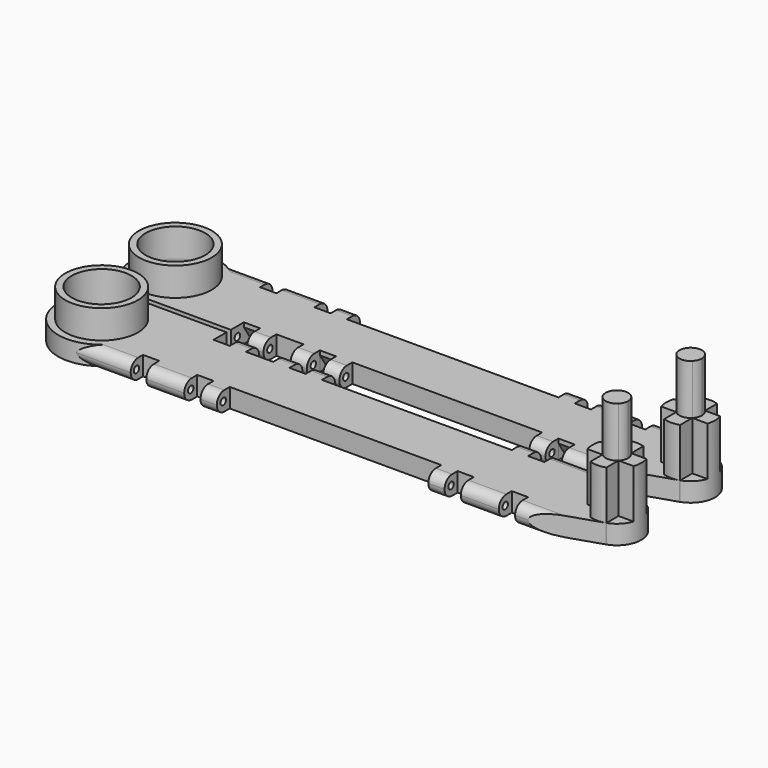
from build123d import *

# Parameters (mm, degrees)
F0_R      = 13.4
F0_R_2    = 11
F0_W      = 6
F0_H      = 6
F1_DEPTH  = 3.5
F2_DEPTH  = 21.5
F3_DEPTH  = 40
F4_DEPTH  = 3.5
F5_R      = 1.25
F6_DEPTH  = 34
F7_DEPTH  = 116
F8_R      = 1.25
F9_DEPTH  = 38
F10_DEPTH = 116
F11_R     = 3.49999
F12_W     = 6
F12_H     = 10
F13_ANGLE = 57
F14_DEPTH = 14


# Not quite as in the source:
# - a fillet or chamfer is up to 0.001 mm smaller than in the source, because OpenCascade refuses the exact size
# - a feature names something its author has since deleted; it is built from what else it names


with BuildPart() as f1:
    # F0 (on Top) → F1 (new body)
    with BuildSketch(Plane.XY):
        with BuildLine():
            ThreePointArc((86.4885738563, -2.925), (86, 0), (86.4885738563, 2.925))
            ThreePointArc((86.4885738563, 2.925), (87.9140641886, 5.5488299377), (90.1195766297, 7.561842879))
            Line((90.1195766297, 7.561842879), (75, 12.5))
            Line((75, 12.5), (73.75, 12.5))
            Line((73.75, 12.5), (73.75, 6.5))
            Line((73.75, 6.5), (-80.3798084828, 6.5))
            ThreePointArc((-80.3798084828, 6.5), (-79.3487530165, 3.3224189775), (-79, 0))
            ThreePointArc((-79, 0), (-80.5812643612, -6.9354208653), (-85.0125078223, -12.5))
            Line((-85.0125078223, -12.5), (-65.25, -12.5))
            Line((-65.25, -12.5), (-65.25, -6.5))
            Line((-65.25, -6.5), (63.75, -6.5))
            Line((63.75, -6.5), (63.75, -12.5))
            Line((63.75, -12.5), (75, -12.5))
            Line((75, -12.5), (90.1195766297, -7.561842879))
            ThreePointArc((90.1195766297, -7.561842879), (87.9140641886, -5.5488299377), (86.4885738563, -2.925))
        make_face()
        with BuildLine():
            ThreePointArc((92.0560443278, 8.5048883003), (94.9210029481, 8.999653297), (97.7942053305, 8.5552566631))
            Line((97.7942053305, 8.5552566631), (75, 16))
            Line((75, 16), (70.25, 16))
            Line((70.25, 16), (70.25, 10))
            Line((70.25, 10), (64.25, 10))
            Line((64.25, 10), (64.25, 16))
            Line((64.25, 16), (50.25, 16))
            Line((50.25, 16), (50.25, 10))
            Line((50.25, 10), (44.25, 10))
            Line((44.25, 10), (44.25, 16))
            Line((44.25, 16), (38.25, 16))
            Line((38.25, 16), (38.25, 10))
            Line((38.25, 10), (-33.75, 10))
            Line((-33.75, 10), (-39.75, 10))
            Line((-39.75, 10), (-39.75, 16))
            Line((-39.75, 16), (-45.75, 16))
            Line((-45.75, 16), (-45.75, 10))
            Line((-45.75, 10), (-51.75, 10))
            Line((-51.75, 10), (-51.75, 16))
            Line((-51.75, 16), (-65.75, 16))
            Line((-65.75, 16), (-65.75, 10))
            Line((-65.75, 10), (-71.75, 10))
            Line((-71.75, 10), (-71.75, 15.6664450339))
            Line((-71.75, 15.6664450339), (-91.75, 15.6664450339))
            ThreePointArc((-91.75, 15.6664450339), (-84.9579949783, 12.4562488392), (-80.3798084828, 6.5))
            Line((-80.3798084828, 6.5), (73.75, 6.5))
            Line((73.75, 6.5), (73.75, 12.5))
            Line((73.75, 12.5), (75, 12.5))
            Line((75, 12.5), (90.1195766297, 7.561842879))
            ThreePointArc((90.1195766297, 7.561842879), (91.0594974284, 8.0915041545), (92.0560443278, 8.5048883003))
        make_face()
        with BuildLine():
            ThreePointArc((-79, 0), (-79.3487530165, 3.3224189775), (-80.3798084828, 6.5))
            ThreePointArc((-80.3798084828, 6.5), (-84.9579949783, 12.4562488392), (-91.75, 15.6664450339))
            ThreePointArc((-91.75, 15.6664450339), (-110.9163928159, 1.6335359588), (-95, -16))
            ThreePointArc((-95, -16), (-89.7084973779, -15.0996688705), (-85.0125078223, -12.5))
            ThreePointArc((-85.0125078223, -12.5), (-80.5812643612, -6.9354208653), (-79, 0))
        make_face()
        with Locations((-95, 0)):
            Circle(F0_R, mode=Mode.SUBTRACT)
        with BuildLine():
            Line((75, -16), (97.7942053305, -8.5552566631))
            ThreePointArc((97.7942053305, -8.5552566631), (94.9210029481, -8.999653297), (92.0560443278, -8.5048883003))
            ThreePointArc((92.0560443278, -8.5048883003), (91.0594974284, -8.0915041545), (90.1195766297, -7.561842879))
            Line((90.1195766297, -7.561842879), (75, -12.5))
            Line((75, -12.5), (63.75, -12.5))
            Line((63.75, -12.5), (63.75, -6.5))
            Line((63.75, -6.5), (-65.25, -6.5))
            Line((-65.25, -6.5), (-65.25, -12.5))
            Line((-65.25, -12.5), (-85.0125078223, -12.5))
            ThreePointArc((-85.0125078223, -12.5), (-89.7084973779, -15.0996688705), (-95, -16))
            Line((-95, -16), (-61.75, -16))
            Line((-61.75, -16), (-61.75, -10))
            Line((-61.75, -10), (-55.75, -10))
            Line((-55.75, -10), (-55.75, -16))
            Line((-55.75, -16), (-49.75, -16))
            Line((-49.75, -16), (-49.75, -10))
            Line((-49.75, -10), (-43.75, -10))
            Line((-43.75, -10), (-39.75, -10))
            Line((-39.75, -10), (-33.75, -10))
            Line((-33.75, -10), (-27.75, -10))
            Line((-27.75, -10), (-21.75, -10))
            Line((-21.75, -10), (48.25, -10))
            Line((48.25, -10), (48.25, -16))
            Line((48.25, -16), (54.25, -16))
            Line((54.25, -16), (54.25, -10))
            Line((54.25, -10), (60.25, -10))
            Line((60.25, -10), (60.25, -16))
            Line((60.25, -16), (75, -16))
        make_face()
        with Locations((-95, 0)):
            Circle(F0_R)
        with Locations((-95, 0)):
            Circle(F0_R_2, mode=Mode.SUBTRACT)
        with Locations((-36.75, -13)):
            Rectangle(F0_W, F0_H)
        with Locations((-24.75, -13)):
            Rectangle(F0_W, F0_H)
        with BuildLine():
            ThreePointArc((90.3422779173, -2.925), (89.5, 0), (90.3422779173, 2.925))
            Line((90.3422779173, 2.925), (86.4885738563, 2.925))
            ThreePointArc((86.4885738563, 2.925), (86, 0), (86.4885738563, -2.925))
            Line((86.4885738563, -2.925), (90.3422779173, -2.925))
        make_face()
        with BuildLine():
            Line((103.5114261437, 2.925), (99.6577220827, 2.925))
            ThreePointArc((99.6577220827, 2.925), (100.285237528, 1.5219278145), (100.5, 0))
            ThreePointArc((100.5, 0), (100.285237528, -1.5219278145), (99.6577220827, -2.925))
            Line((99.6577220827, -2.925), (103.5114261437, -2.925))
            ThreePointArc((103.5114261437, -2.925), (103.8770162581, -1.4827617318), (104, 0))
            ThreePointArc((104, 0), (103.8770162581, 1.4827617318), (103.5114261437, 2.925))
        make_face()
        with BuildLine():
            Line((103.5114261437, -2.925), (99.6577220827, -2.925))
            ThreePointArc((99.6577220827, -2.925), (98.8970031473, -3.8811553009), (97.9439556722, -4.6457641998))
            Line((97.9439556722, -4.6457641998), (97.9439556722, -8.5048883003))
            ThreePointArc((97.9439556722, -8.5048883003), (101.3710463425, -6.3568678216), (103.5114261437, -2.925))
        make_face()
        with BuildLine():
            Line((97.9439556722, 8.5048883003), (97.9439556722, 4.6457641998))
            ThreePointArc((97.9439556722, 4.6457641998), (98.8970031473, 3.8811553009), (99.6577220827, 2.925))
            Line((99.6577220827, 2.925), (103.5114261437, 2.925))
            ThreePointArc((103.5114261437, 2.925), (101.3710463425, 6.3568678216), (97.9439556722, 8.5048883003))
        make_face()
        with BuildLine():
            Line((97.9439556722, -8.5048883003), (97.9439556722, -4.6457641998))
            ThreePointArc((97.9439556722, -4.6457641998), (97.4047291369, -4.9464409203), (96.8352012857, -5.1847889293))
            Line((96.8352012857, -5.1847889293), (92.0560443278, -6.876413239))
            Line((92.0560443278, -6.876413239), (92.0560443278, -8.5048883003))
            ThreePointArc((92.0560443278, -8.5048883003), (94.9210029481, -8.999653297), (97.7942053305, -8.5552566631))
            ThreePointArc((97.7942053305, -8.5552566631), (97.8691910299, -8.5304010945), (97.9439556722, -8.5048883003))
        make_face()
        with BuildLine():
            ThreePointArc((96.8352012857, 5.1847889293), (97.4047291369, 4.9464409203), (97.9439556722, 4.6457641998))
            Line((97.9439556722, 4.6457641998), (97.9439556722, 8.5048883003))
            ThreePointArc((97.9439556722, 8.5048883003), (97.8691910299, 8.5304010945), (97.7942053305, 8.5552566631))
            ThreePointArc((97.7942053305, 8.5552566631), (94.9210029481, 8.999653297), (92.0560443278, 8.5048883003))
            Line((92.0560443278, 8.5048883003), (92.0560443278, 6.876413239))
            Line((92.0560443278, 6.876413239), (96.8352012857, 5.1847889293))
        make_face()
        with BuildLine():
            Line((92.0560443278, -6.876413239), (92.0560443278, -4.6457641998))
            ThreePointArc((92.0560443278, -4.6457641998), (91.1029968527, -3.8811553009), (90.3422779173, -2.925))
            Line((90.3422779173, -2.925), (86.4885738563, -2.925))
            ThreePointArc((86.4885738563, -2.925), (87.9140641886, -5.5488299377), (90.1195766297, -7.561842879))
            Line((90.1195766297, -7.561842879), (92.0560443278, -6.876413239))
        make_face()
        with BuildLine():
            ThreePointArc((90.3422779173, 2.925), (91.1029968527, 3.8811553009), (92.0560443278, 4.6457641998))
            Line((92.0560443278, 4.6457641998), (92.0560443278, 6.876413239))
            Line((92.0560443278, 6.876413239), (90.1195766297, 7.561842879))
            ThreePointArc((90.1195766297, 7.561842879), (87.9140641886, 5.5488299377), (86.4885738563, 2.925))
            Line((86.4885738563, 2.925), (90.3422779173, 2.925))
        make_face()
        with BuildLine():
            Line((97.9439556722, -4.6457641998), (97.9439556722, -2.925))
            ThreePointArc((97.9439556722, -2.925), (95, -4.15), (92.0560443278, -2.925))
            Line((92.0560443278, -2.925), (92.0560443278, -4.6457641998))
            ThreePointArc((92.0560443278, -4.6457641998), (94.3835821327, -5.465348023), (96.8352012857, -5.1847889293))
            ThreePointArc((96.8352012857, -5.1847889293), (97.4047291369, -4.9464409203), (97.9439556722, -4.6457641998))
        make_face()
        with BuildLine():
            ThreePointArc((92.0560443278, 2.925), (95, 4.15), (97.9439556722, 2.925))
            Line((97.9439556722, 2.925), (97.9439556722, 4.6457641998))
            ThreePointArc((97.9439556722, 4.6457641998), (97.4047291369, 4.9464409203), (96.8352012857, 5.1847889293))
            ThreePointArc((96.8352012857, 5.1847889293), (94.3835821327, 5.465348023), (92.0560443278, 4.6457641998))
            Line((92.0560443278, 4.6457641998), (92.0560443278, 2.925))
        make_face()
        with BuildLine():
            Line((92.0560443278, 6.876413239), (92.0560443278, 4.6457641998))
            ThreePointArc((92.0560443278, 4.6457641998), (94.3835821327, 5.465348023), (96.8352012857, 5.1847889293))
            Line((96.8352012857, 5.1847889293), (92.0560443278, 6.876413239))
        make_face()
        with BuildLine():
            ThreePointArc((96.8352012857, -5.1847889293), (94.3835821327, -5.465348023), (92.0560443278, -4.6457641998))
            Line((92.0560443278, -4.6457641998), (92.0560443278, -6.876413239))
            Line((92.0560443278, -6.876413239), (96.8352012857, -5.1847889293))
        make_face()
        with BuildLine():
            Line((92.0560443278, -4.6457641998), (92.0560443278, -2.925))
            Line((92.0560443278, -2.925), (90.3422779173, -2.925))
            ThreePointArc((90.3422779173, -2.925), (91.1029968527, -3.8811553009), (92.0560443278, -4.6457641998))
        make_face()
        with BuildLine():
            Line((99.6577220827, -2.925), (97.9439556722, -2.925))
            Line((97.9439556722, -2.925), (97.9439556722, -4.6457641998))
            ThreePointArc((97.9439556722, -4.6457641998), (98.8970031473, -3.8811553009), (99.6577220827, -2.925))
        make_face()
        with BuildLine():
            Line((97.9439556722, 4.6457641998), (97.9439556722, 2.925))
            Line((97.9439556722, 2.925), (99.6577220827, 2.925))
            ThreePointArc((99.6577220827, 2.925), (98.8970031473, 3.8811553009), (97.9439556722, 4.6457641998))
        make_face()
        with BuildLine():
            Line((90.3422779173, 2.925), (92.0560443278, 2.925))
            Line((92.0560443278, 2.925), (92.0560443278, 4.6457641998))
            ThreePointArc((92.0560443278, 4.6457641998), (91.1029968527, 3.8811553009), (90.3422779173, 2.925))
        make_face()
        with BuildLine():
            Line((92.0560443278, -8.5048883003), (92.0560443278, -6.876413239))
            Line((92.0560443278, -6.876413239), (90.1195766297, -7.561842879))
            ThreePointArc((90.1195766297, -7.561842879), (91.0594974284, -8.0915041545), (92.0560443278, -8.5048883003))
        make_face()
        with BuildLine():
            Line((90.1195766297, 7.561842879), (92.0560443278, 6.876413239))
            Line((92.0560443278, 6.876413239), (92.0560443278, 8.5048883003))
            ThreePointArc((92.0560443278, 8.5048883003), (91.0594974284, 8.0915041545), (90.1195766297, 7.561842879))
        make_face()
    extrude(amount=F1_DEPTH)

    # F0 (on Top) → F2 (join)
    with BuildSketch(Plane.XY):
        with BuildLine():
            ThreePointArc((97.9439556722, -2.925), (98.8366597477, -1.5819424706), (99.15, 0))
            ThreePointArc((99.15, 0), (98.8366597477, 1.5819424706), (97.9439556722, 2.925))
            ThreePointArc((97.9439556722, 2.925), (95, 4.15), (92.0560443278, 2.925))
            ThreePointArc((92.0560443278, 2.925), (90.85, 0), (92.0560443278, -2.925))
            ThreePointArc((92.0560443278, -2.925), (95, -4.15), (97.9439556722, -2.925))
        make_face()
        with BuildLine():
            ThreePointArc((92.0560443278, 2.925), (95, 4.15), (97.9439556722, 2.925))
            Line((97.9439556722, 2.925), (97.9439556722, 4.6457641998))
            ThreePointArc((97.9439556722, 4.6457641998), (97.4047291369, 4.9464409203), (96.8352012857, 5.1847889293))
            ThreePointArc((96.8352012857, 5.1847889293), (94.3835821327, 5.465348023), (92.0560443278, 4.6457641998))
            Line((92.0560443278, 4.6457641998), (92.0560443278, 2.925))
        make_face()
        with BuildLine():
            ThreePointArc((92.0560443278, -2.925), (90.85, 0), (92.0560443278, 2.925))
            Line((92.0560443278, 2.925), (90.3422779173, 2.925))
            ThreePointArc((90.3422779173, 2.925), (89.5, 0), (90.3422779173, -2.925))
            Line((90.3422779173, -2.925), (92.0560443278, -2.925))
        make_face()
        with BuildLine():
            Line((97.9439556722, -4.6457641998), (97.9439556722, -2.925))
            ThreePointArc((97.9439556722, -2.925), (95, -4.15), (92.0560443278, -2.925))
            Line((92.0560443278, -2.925), (92.0560443278, -4.6457641998))
            ThreePointArc((92.0560443278, -4.6457641998), (94.3835821327, -5.465348023), (96.8352012857, -5.1847889293))
            ThreePointArc((96.8352012857, -5.1847889293), (97.4047291369, -4.9464409203), (97.9439556722, -4.6457641998))
        make_face()
        with BuildLine():
            ThreePointArc((97.9439556722, 2.925), (98.8366597477, 1.5819424706), (99.15, 0))
            ThreePointArc((99.15, 0), (98.8366597477, -1.5819424706), (97.9439556722, -2.925))
            Line((97.9439556722, -2.925), (99.6577220827, -2.925))
            ThreePointArc((99.6577220827, -2.925), (100.285237528, -1.5219278145), (100.5, 0))
            ThreePointArc((100.5, 0), (100.285237528, 1.5219278145), (99.6577220827, 2.925))
            Line((99.6577220827, 2.925), (97.9439556722, 2.925))
        make_face()
        with BuildLine():
            Line((92.0560443278, 6.876413239), (92.0560443278, 4.6457641998))
            ThreePointArc((92.0560443278, 4.6457641998), (94.3835821327, 5.465348023), (96.8352012857, 5.1847889293))
            Line((96.8352012857, 5.1847889293), (92.0560443278, 6.876413239))
        make_face()
        with BuildLine():
            ThreePointArc((96.8352012857, 5.1847889293), (97.4047291369, 4.9464409203), (97.9439556722, 4.6457641998))
            Line((97.9439556722, 4.6457641998), (97.9439556722, 8.5048883003))
            ThreePointArc((97.9439556722, 8.5048883003), (97.8691910299, 8.5304010945), (97.7942053305, 8.5552566631))
            ThreePointArc((97.7942053305, 8.5552566631), (94.9210029481, 8.999653297), (92.0560443278, 8.5048883003))
            Line((92.0560443278, 8.5048883003), (92.0560443278, 6.876413239))
            Line((92.0560443278, 6.876413239), (96.8352012857, 5.1847889293))
        make_face()
        with BuildLine():
            Line((97.9439556722, -8.5048883003), (97.9439556722, -4.6457641998))
            ThreePointArc((97.9439556722, -4.6457641998), (97.4047291369, -4.9464409203), (96.8352012857, -5.1847889293))
            Line((96.8352012857, -5.1847889293), (92.0560443278, -6.876413239))
            Line((92.0560443278, -6.876413239), (92.0560443278, -8.5048883003))
            ThreePointArc((92.0560443278, -8.5048883003), (94.9210029481, -8.999653297), (97.7942053305, -8.5552566631))
            ThreePointArc((97.7942053305, -8.5552566631), (97.8691910299, -8.5304010945), (97.9439556722, -8.5048883003))
        make_face()
        with BuildLine():
            ThreePointArc((96.8352012857, -5.1847889293), (94.3835821327, -5.465348023), (92.0560443278, -4.6457641998))
            Line((92.0560443278, -4.6457641998), (92.0560443278, -6.876413239))
            Line((92.0560443278, -6.876413239), (96.8352012857, -5.1847889293))
        make_face()
        with BuildLine():
            ThreePointArc((90.3422779173, -2.925), (89.5, 0), (90.3422779173, 2.925))
            Line((90.3422779173, 2.925), (86.4885738563, 2.925))
            ThreePointArc((86.4885738563, 2.925), (86, 0), (86.4885738563, -2.925))
            Line((86.4885738563, -2.925), (90.3422779173, -2.925))
        make_face()
        with BuildLine():
            Line((103.5114261437, 2.925), (99.6577220827, 2.925))
            ThreePointArc((99.6577220827, 2.925), (100.285237528, 1.5219278145), (100.5, 0))
            ThreePointArc((100.5, 0), (100.285237528, -1.5219278145), (99.6577220827, -2.925))
            Line((99.6577220827, -2.925), (103.5114261437, -2.925))
            ThreePointArc((103.5114261437, -2.925), (103.8770162581, -1.4827617318), (104, 0))
            ThreePointArc((104, 0), (103.8770162581, 1.4827617318), (103.5114261437, 2.925))
        make_face()
    extrude(amount=F2_DEPTH)

    # F0 (on Top) → F3 (join)
    with BuildSketch(Plane.XY):
        with BuildLine():
            ThreePointArc((97.9439556722, -2.925), (98.8366597477, -1.5819424706), (99.15, 0))
            ThreePointArc((99.15, 0), (98.8366597477, 1.5819424706), (97.9439556722, 2.925))
            ThreePointArc((97.9439556722, 2.925), (95, 4.15), (92.0560443278, 2.925))
            ThreePointArc((92.0560443278, 2.925), (90.85, 0), (92.0560443278, -2.925))
            ThreePointArc((92.0560443278, -2.925), (95, -4.15), (97.9439556722, -2.925))
        make_face()
    extrude(amount=F3_DEPTH)

    # F0 (on Top) → F4 (join)
    with BuildSketch(Plane.XY):
        with BuildLine():
            ThreePointArc((92.0560443278, 8.5048883003), (94.9210029481, 8.999653297), (97.7942053305, 8.5552566631))
            Line((97.7942053305, 8.5552566631), (75, 16))
            Line((75, 16), (70.25, 16))
            Line((70.25, 16), (70.25, 10))
            Line((70.25, 10), (64.25, 10))
            Line((64.25, 10), (64.25, 16))
            Line((64.25, 16), (50.25, 16))
            Line((50.25, 16), (50.25, 10))
            Line((50.25, 10), (44.25, 10))
            Line((44.25, 10), (44.25, 16))
            Line((44.25, 16), (38.25, 16))
            Line((38.25, 16), (38.25, 10))
            Line((38.25, 10), (-33.75, 10))
            Line((-33.75, 10), (-39.75, 10))
            Line((-39.75, 10), (-39.75, 16))
            Line((-39.75, 16), (-45.75, 16))
            Line((-45.75, 16), (-45.75, 10))
            Line((-45.75, 10), (-51.75, 10))
            Line((-51.75, 10), (-51.75, 16))
            Line((-51.75, 16), (-65.75, 16))
            Line((-65.75, 16), (-65.75, 10))
            Line((-65.75, 10), (-71.75, 10))
            Line((-71.75, 10), (-71.75, 15.6664450339))
            Line((-71.75, 15.6664450339), (-91.75, 15.6664450339))
            ThreePointArc((-91.75, 15.6664450339), (-84.9579949783, 12.4562488392), (-80.3798084828, 6.5))
            Line((-80.3798084828, 6.5), (73.75, 6.5))
            Line((73.75, 6.5), (73.75, 12.5))
            Line((73.75, 12.5), (75, 12.5))
            Line((75, 12.5), (90.1195766297, 7.561842879))
            ThreePointArc((90.1195766297, 7.561842879), (91.0594974284, 8.0915041545), (92.0560443278, 8.5048883003))
        make_face()
        with BuildLine():
            ThreePointArc((-79, 0), (-79.3487530165, 3.3224189775), (-80.3798084828, 6.5))
            ThreePointArc((-80.3798084828, 6.5), (-84.9579949783, 12.4562488392), (-91.75, 15.6664450339))
            ThreePointArc((-91.75, 15.6664450339), (-110.9163928159, 1.6335359588), (-95, -16))
            ThreePointArc((-95, -16), (-89.7084973779, -15.0996688705), (-85.0125078223, -12.5))
            ThreePointArc((-85.0125078223, -12.5), (-80.5812643612, -6.9354208653), (-79, 0))
        make_face()
        with Locations((-95, 0)):
            Circle(F0_R, mode=Mode.SUBTRACT)
        with BuildLine():
            Line((75, -16), (97.7942053305, -8.5552566631))
            ThreePointArc((97.7942053305, -8.5552566631), (94.9210029481, -8.999653297), (92.0560443278, -8.5048883003))
            ThreePointArc((92.0560443278, -8.5048883003), (91.0594974284, -8.0915041545), (90.1195766297, -7.561842879))
            Line((90.1195766297, -7.561842879), (75, -12.5))
            Line((75, -12.5), (63.75, -12.5))
            Line((63.75, -12.5), (63.75, -6.5))
            Line((63.75, -6.5), (-65.25, -6.5))
            Line((-65.25, -6.5), (-65.25, -12.5))
            Line((-65.25, -12.5), (-85.0125078223, -12.5))
            ThreePointArc((-85.0125078223, -12.5), (-89.7084973779, -15.0996688705), (-95, -16))
            Line((-95, -16), (-61.75, -16))
            Line((-61.75, -16), (-61.75, -10))
            Line((-61.75, -10), (-55.75, -10))
            Line((-55.75, -10), (-55.75, -16))
            Line((-55.75, -16), (-49.75, -16))
            Line((-49.75, -16), (-49.75, -10))
            Line((-49.75, -10), (-43.75, -10))
            Line((-43.75, -10), (-39.75, -10))
            Line((-39.75, -10), (-33.75, -10))
            Line((-33.75, -10), (-27.75, -10))
            Line((-27.75, -10), (-21.75, -10))
            Line((-21.75, -10), (48.25, -10))
            Line((48.25, -10), (48.25, -16))
            Line((48.25, -16), (54.25, -16))
            Line((54.25, -16), (54.25, -10))
            Line((54.25, -10), (60.25, -10))
            Line((60.25, -10), (60.25, -16))
            Line((60.25, -16), (75, -16))
        make_face()
        with Locations((-95, 0)):
            Circle(F0_R)
        with Locations((-95, 0)):
            Circle(F0_R_2, mode=Mode.SUBTRACT)
        with Locations((-24.75, -13)):
            Rectangle(F0_W, F0_H)
        with Locations((-36.75, -13)):
            Rectangle(F0_W, F0_H)
        with BuildLine():
            Line((103.5114261437, 2.925), (99.6577220827, 2.925))
            ThreePointArc((99.6577220827, 2.925), (100.285237528, 1.5219278145), (100.5, 0))
            ThreePointArc((100.5, 0), (100.285237528, -1.5219278145), (99.6577220827, -2.925))
            Line((99.6577220827, -2.925), (103.5114261437, -2.925))
            ThreePointArc((103.5114261437, -2.925), (103.8770162581, -1.4827617318), (104, 0))
            ThreePointArc((104, 0), (103.8770162581, 1.4827617318), (103.5114261437, 2.925))
        make_face()
        with BuildLine():
            Line((103.5114261437, -2.925), (99.6577220827, -2.925))
            ThreePointArc((99.6577220827, -2.925), (98.8970031473, -3.8811553009), (97.9439556722, -4.6457641998))
            Line((97.9439556722, -4.6457641998), (97.9439556722, -8.5048883003))
            ThreePointArc((97.9439556722, -8.5048883003), (101.3710463425, -6.3568678216), (103.5114261437, -2.925))
        make_face()
        with BuildLine():
            Line((97.9439556722, 8.5048883003), (97.9439556722, 4.6457641998))
            ThreePointArc((97.9439556722, 4.6457641998), (98.8970031473, 3.8811553009), (99.6577220827, 2.925))
            Line((99.6577220827, 2.925), (103.5114261437, 2.925))
            ThreePointArc((103.5114261437, 2.925), (101.3710463425, 6.3568678216), (97.9439556722, 8.5048883003))
        make_face()
        with BuildLine():
            Line((97.9439556722, -8.5048883003), (97.9439556722, -4.6457641998))
            ThreePointArc((97.9439556722, -4.6457641998), (97.4047291369, -4.9464409203), (96.8352012857, -5.1847889293))
            Line((96.8352012857, -5.1847889293), (92.0560443278, -6.876413239))
            Line((92.0560443278, -6.876413239), (92.0560443278, -8.5048883003))
            ThreePointArc((92.0560443278, -8.5048883003), (94.9210029481, -8.999653297), (97.7942053305, -8.5552566631))
            ThreePointArc((97.7942053305, -8.5552566631), (97.8691910299, -8.5304010945), (97.9439556722, -8.5048883003))
        make_face()
        with BuildLine():
            ThreePointArc((96.8352012857, 5.1847889293), (97.4047291369, 4.9464409203), (97.9439556722, 4.6457641998))
            Line((97.9439556722, 4.6457641998), (97.9439556722, 8.5048883003))
            ThreePointArc((97.9439556722, 8.5048883003), (97.8691910299, 8.5304010945), (97.7942053305, 8.5552566631))
            ThreePointArc((97.7942053305, 8.5552566631), (94.9210029481, 8.999653297), (92.0560443278, 8.5048883003))
            Line((92.0560443278, 8.5048883003), (92.0560443278, 6.876413239))
            Line((92.0560443278, 6.876413239), (96.8352012857, 5.1847889293))
        make_face()
        with BuildLine():
            Line((92.0560443278, -8.5048883003), (92.0560443278, -6.876413239))
            Line((92.0560443278, -6.876413239), (90.1195766297, -7.561842879))
            ThreePointArc((90.1195766297, -7.561842879), (91.0594974284, -8.0915041545), (92.0560443278, -8.5048883003))
        make_face()
        with BuildLine():
            Line((90.1195766297, 7.561842879), (92.0560443278, 6.876413239))
            Line((92.0560443278, 6.876413239), (92.0560443278, 8.5048883003))
            ThreePointArc((92.0560443278, 8.5048883003), (91.0594974284, 8.0915041545), (90.1195766297, 7.561842879))
        make_face()
    extrude(amount=-F4_DEPTH)

    # F5 (on face) → F6 (cut)
    with BuildSketch(Plane.YZ.offset(-49.75)):
        with Locations((-13, 0)):
            Circle(F5_R)
    extrude(amount=-F6_DEPTH, mode=Mode.SUBTRACT)

    # F5 (on face) → F7 (cut)
    with BuildSketch(Plane.YZ.offset(-49.75)):
        with Locations((-13, 0)):
            Circle(F5_R)
    extrude(amount=F7_DEPTH, mode=Mode.SUBTRACT)

    # F8 (on face) → F9 (cut)
    with BuildSketch(Plane(origin=(38.25, 0, 0), x_dir=(0, -1, 0), z_dir=(-1, 0, 0))):
        with Locations((-13, 0)):
            Circle(F8_R)
    extrude(amount=-F9_DEPTH, mode=Mode.SUBTRACT)

    # F8 (on face) → F10 (cut)
    with BuildSketch(Plane(origin=(38.25, 0, 0), x_dir=(0, -1, 0), z_dir=(-1, 0, 0))):
        with Locations((-13, 0)):
            Circle(F8_R)
    extrude(amount=F10_DEPTH, mode=Mode.SUBTRACT)

    # F11 (radius 3.5 in the source; OpenCascade refuses exactly that, so slightly less here)
    f11_edges = [f1.edges().sort_by_distance(p)[0] for p in [
        (41.25, 16, 3.5),
        (41.25, 16, -3.5),
        (57.25, 16, 3.5),
        (57.25, 16, -3.5),
        (72.625, 16, 3.5),
        (72.625, 16, -3.5),
        (67.625, -16, -3.5),
        (51.25, -16, -3.5),
        (-81.75, 15.666445, -3.5),
        (-81.75, 15.666445, 3.5),
        (-58.75, 16, -3.5),
        (-58.75, 16, 3.5),
        (-42.75, 16, -3.5),
        (-42.75, 16, 3.5),
        (-52.75, -16, 3.5),
        (-52.75, -16, -3.5),
        (51.25, -16, 3.5),
        (67.625, -16, 3.5),
        (-24.75, -16, -3.5),
        (-36.75, -16, -3.5),
        (-24.75, -16, 3.5),
        (-36.75, -16, 3.5),
    ]]
    fillet(f11_edges, radius=F11_R)

    # F12 (on face) → F13 (revolve, cut)
    with BuildSketch(Plane(origin=(0, 0, -3.5), x_dir=(1, 0, 0), z_dir=(0, 0, -1))):
        Polygon((54.25, 6.5), (60.25, 6.5), (60.25, 16.6681855917), (54.25, 16.6681855917), (54.25, 16.5), align=None)
        with Locations((-58.75, 11.5)):
            Rectangle(F12_W, F12_H)
        with Locations((-30.75, 11.5)):
            Rectangle(F12_W, F12_H)
    revolve(axis=Axis((-0.75, -6.5, -3.5), (-1, 0, 0)), revolution_arc=F13_ANGLE, mode=Mode.SUBTRACT)

    # F0 (on Top) → F14 (join)
    with BuildSketch(Plane.XY):
        with Locations((-95, 0)):
            Circle(F0_R)
        with Locations((-95, 0)):
            Circle(F0_R_2, mode=Mode.SUBTRACT)
    extrude(amount=F14_DEPTH)


with BuildPart() as f16_1:
    # F16: instance of F1
    add(f1.part.mirror(Plane.XZ.offset(17)))


solid = Compound([f1.part, f16_1.part])
